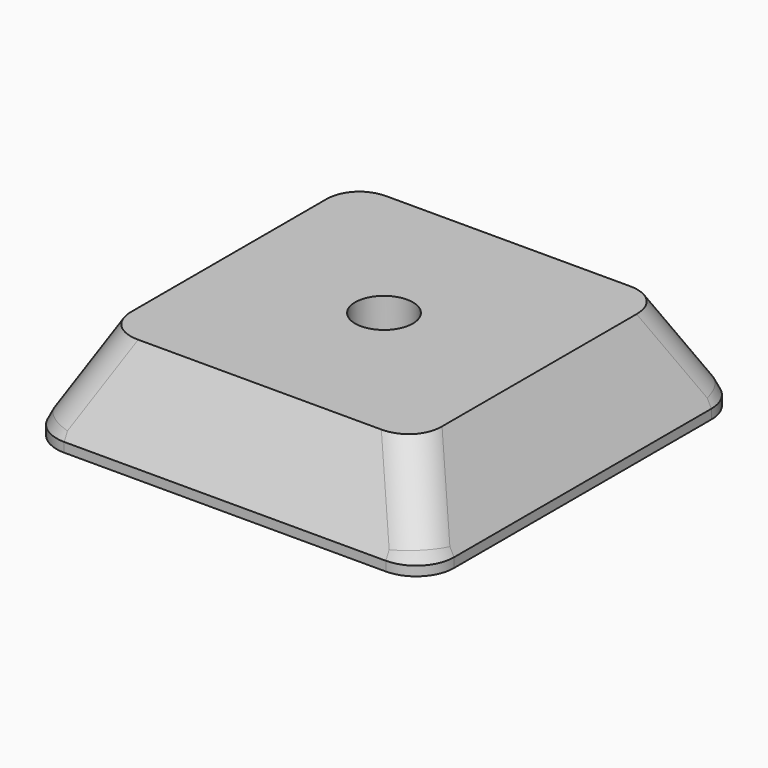
from build123d import *

# Parameters (mm, degrees)
F1_DEPTH    = 1
F2_DEPTH    = 9
F2_TAPER    = 27
F3_T1_DEPTH = 17.6431556895
F3_T3_DEPTH = 17.6431556895
F3_T5_DEPTH = 17.6431556895
F3_T7_DEPTH = 17.6431556895
F4_R        = 18
F5_DEPTH    = 6
F5_TAPER    = 27
F6_R        = 3.05
F7_DEPTH    = 4.0010001


# Not quite as in the source:
# - a fillet or chamfer that OpenCascade refuses, or shapes differently, is made with other operations: its cross-section is extruded or revolved along the edge and cut away or added


with BuildPart() as f1:
    # F0 (on Top) → F1 (new body)
    with BuildSketch(Plane.XY):
        with BuildLine():
            Line((-17, -21), (17, -21))
            ThreePointArc((17, -21), (19.8284271247, -19.8284271247), (21, -17))
            Line((21, -17), (21, 17))
            ThreePointArc((21, 17), (19.8284271247, 19.8284271247), (17, 21))
            Line((17, 21), (-17, 21))
            ThreePointArc((-17, 21), (-19.8284271247, 19.8284271247), (-21, 17))
            Line((-21, 17), (-21, -17))
            ThreePointArc((-21, -17), (-19.8284271247, -19.8284271247), (-17, -21))
        make_face()
    extrude(amount=F1_DEPTH)

    # F1_face (on face) → F2 (join)
    with BuildSketch(Plane.XY.offset(1)):
        with BuildLine():
            Line((-17, -21), (17, -21))
            ThreePointArc((17, -21), (19.8284271247, -19.8284271247), (21, -17))
            Line((21, -17), (21, 17))
            ThreePointArc((21, 17), (19.8284271247, 19.8284271247), (17, 21))
            Line((17, 21), (-17, 21))
            ThreePointArc((-17, 21), (-19.8284271247, 19.8284271247), (-21, 17))
            Line((-21, 17), (-21, -17))
            ThreePointArc((-21, -17), (-19.8284271247, -19.8284271247), (-17, -21))
        make_face()
    extrude(amount=F2_DEPTH, taper=F2_TAPER)

    # F3: fillet of radius 4 on 4 edges, made by hand

    # F3_s2 → F3_t1 (cut)
    with BuildSketch(Plane(origin=(-6.1956825311, -6.1956825311, -12.1597116243), x_dir=(-0.7071067812, 0.7071067812, 0), z_dir=(0.4133841097, 0.4133841097, 0.8113119965))):
        with BuildLine():
            ThreePointArc((-2.5201470213, 22.6347249075), (0, 23.5284636515), (2.5201470213, 22.6347249075))
            Line((2.5201470213, 22.6347249075), (0, 24.6793504189))
            Line((0, 24.6793504189), (-2.5201470213, 22.6347249075))
        make_face()
    extrude(amount=F3_T1_DEPTH, mode=Mode.SUBTRACT)

    # F3_s4 → F3_t3 (cut)
    with BuildSketch(Plane(origin=(6.1956825311, -6.1956825311, -12.1597116243), x_dir=(-0.7071067812, -0.7071067812, 0), z_dir=(-0.4133841097, 0.4133841097, 0.8113119965))):
        with BuildLine():
            ThreePointArc((2.5201470213, 22.6347249075), (0, 23.5284636515), (-2.5201470213, 22.6347249075))
            Line((-2.5201470213, 22.6347249075), (0, 24.6793504189))
            Line((0, 24.6793504189), (2.5201470213, 22.6347249075))
        make_face()
    extrude(amount=F3_T3_DEPTH, mode=Mode.SUBTRACT)

    # F3_s6 → F3_t5 (cut)
    with BuildSketch(Plane(origin=(-6.1956825311, 6.1956825311, -12.1597116243), x_dir=(0.7071067812, 0.7071067812, 0), z_dir=(0.4133841097, -0.4133841097, 0.8113119965))):
        with BuildLine():
            ThreePointArc((-2.5201470213, 22.6347249075), (0, 23.5284636515), (2.5201470213, 22.6347249075))
            Line((2.5201470213, 22.6347249075), (0, 24.6793504189))
            Line((0, 24.6793504189), (-2.5201470213, 22.6347249075))
        make_face()
    extrude(amount=F3_T5_DEPTH, mode=Mode.SUBTRACT)

    # F3_s8 → F3_t7 (cut)
    with BuildSketch(Plane(origin=(6.1956825311, 6.1956825311, -12.1597116243), x_dir=(0.7071067812, -0.7071067812, 0), z_dir=(-0.4133841097, -0.4133841097, 0.8113119965))):
        with BuildLine():
            ThreePointArc((2.5201470213, 22.6347249075), (0, 23.5284636515), (-2.5201470213, 22.6347249075))
            Line((-2.5201470213, 22.6347249075), (0, 24.6793504189))
            Line((0, 24.6793504189), (2.5201470213, 22.6347249075))
        make_face()
    extrude(amount=F3_T7_DEPTH, mode=Mode.SUBTRACT)

    # F4 (on face) → F5 (cut)
    with BuildSketch(Plane(origin=(0, 0, 0), x_dir=(1, 0, 0), z_dir=(0, 0, -1))):
        Circle(F4_R)
    extrude(amount=-F5_DEPTH, taper=F5_TAPER, mode=Mode.SUBTRACT)

    # F6 (on face) → F7 (cut, through all)
    with BuildSketch(Plane(origin=(0, 0, 6), x_dir=(1, 0, 0), z_dir=(0, 0, -1))):
        Circle(F6_R)
    extrude(amount=-F7_DEPTH, mode=Mode.SUBTRACT)


solid = f1.part
